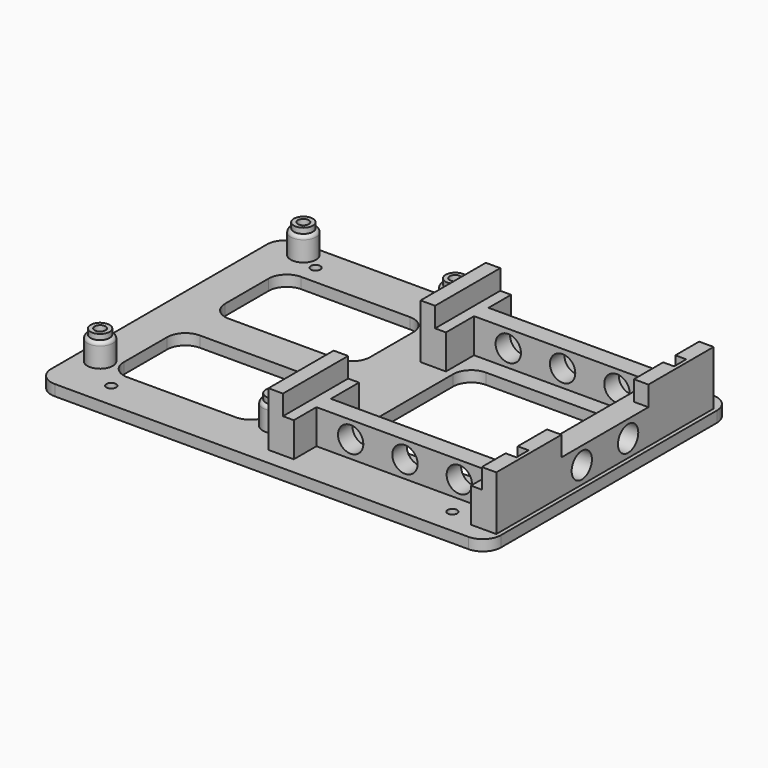
from build123d import *

# Parameters (mm, degrees)
F0_R      = 1.325
F1_DEPTH  = 3
F2_R      = 2.625
F2_R_2    = 1.5
F3_DEPTH  = 8
F4_R      = 3.5
F5_DEPTH  = 6.5
F7_DEPTH  = 7.5
F8_W      = 4
F8_H      = 75
F9_DEPTH  = 10
F10_W     = 4
F10_H     = 75
F11_DEPTH = 10
F13_DEPTH = 10
F14_W     = 30
F14_H     = 17.5
F15_DEPTH = 64.001
F16_W     = 4
F16_H     = 2.5
F17_DEPTH = 79.751
F20_DEPTH = 3.001
F18_W     = 48.9
F18_H     = 5
F21_DEPTH = 7.5
F23_DEPTH = 3.001
F24_W     = 4
F24_H     = 2.5
F25_DEPTH = 79.751
F26_DEPTH = 9.501
F27_W     = 7
F27_H     = 30
F28_DEPTH = 7.5
F30_DEPTH = 2
F31_R     = 3.5
F32_DEPTH = 71.951
F33_R     = 3.5
F34_DEPTH = 123.101


# Not quite as in the source:
# - a fillet or chamfer that OpenCascade refuses, or shapes differently, is made with other operations: its cross-section is extruded or revolved along the edge and cut away or added


with BuildPart() as f1:
    # F0 (on Top) → F1 (new body)
    with BuildSketch(Plane.XY):
        with BuildLine():
            Line((57.1, 42.25), (0, 42.25))
            Line((0, 42.25), (-57.1, 42.25))
            ThreePointArc((-57.1, 42.25), (-60.6355339059, 40.7855339059), (-62.1, 37.25))
            Line((-62.1, 37.25), (-62.1, 0))
            Line((-62.1, 0), (-62.1, -37.25))
            ThreePointArc((-62.1, -37.25), (-60.6355339059, -40.7855339059), (-57.1, -42.25))
            Line((-57.1, -42.25), (0, -42.25))
            Line((0, -42.25), (57.1, -42.25))
            ThreePointArc((57.1, -42.25), (60.6355339059, -40.7855339059), (62.1, -37.25))
            Line((62.1, -37.25), (62.1, 0))
            Line((62.1, 0), (62.1, 37.25))
            ThreePointArc((62.1, 37.25), (60.6355339059, 40.7855339059), (57.1, 42.25))
        make_face()
        with Locations((-47.1, -35.25)):
            Circle(F0_R, mode=Mode.SUBTRACT)
        with Locations((47.1, -35.25)):
            Circle(F0_R, mode=Mode.SUBTRACT)
        with Locations((-47.1, 35.25)):
            Circle(F0_R, mode=Mode.SUBTRACT)
        with Locations((47.1, 35.25)):
            Circle(F0_R, mode=Mode.SUBTRACT)
    extrude(amount=F1_DEPTH)

    # F2 (on face) → F3 (join)
    with BuildSketch(Plane.XY.offset(3)):
        with Locations((-56.1, -27.85)):
            Circle(F2_R)
        with Locations((-56.1, -27.85)):
            Circle(F2_R_2, mode=Mode.SUBTRACT)
        with Locations((-7.71, -27.85)):
            Circle(F2_R)
        with Locations((-7.71, -27.85)):
            Circle(F2_R_2, mode=Mode.SUBTRACT)
        with Locations((-52.86, 38.25)):
            Circle(F2_R)
        with Locations((-52.86, 38.25)):
            Circle(F2_R_2, mode=Mode.SUBTRACT)
        with Locations((-10.95, 38.25)):
            Circle(F2_R)
        with Locations((-10.95, 38.25)):
            Circle(F2_R_2, mode=Mode.SUBTRACT)
    extrude(amount=F3_DEPTH)

    # F4 (on face) → F5 (join)
    with BuildSketch(Plane.XY.offset(3)):
        with Locations((-10.95, 38.25)):
            Circle(F4_R)
        with Locations((-7.71, -27.85)):
            Circle(F4_R)
        with Locations((-56.1, -27.85)):
            Circle(F4_R)
        with Locations((-52.86, 38.25)):
            Circle(F4_R)
    extrude(amount=F5_DEPTH)

    # F6 (on face) → F7 (join)
    with BuildSketch(Plane.XY.offset(3)):
        Polygon((5.1, 37.5), (2.1, 37.5), (-1.9, 37.5), (-1.9, -37.5), (2.1, -37.5), (5.1, -37.5), align=None)
        Polygon((61, 37.5), (57, 37.5), (54, 37.5), (54, -37.5), (57, -37.5), (61, -37.5), align=None)
    extrude(amount=F7_DEPTH)

    # F8 (on face) → F9 (join)
    with BuildSketch(Plane.XY.offset(10.5)):
        with Locations((0.1, 0)):
            Rectangle(F8_W, F8_H)
    extrude(amount=F9_DEPTH)

    # F10 (on face) → F11 (join)
    with BuildSketch(Plane.XY.offset(10.5)):
        with Locations((59, 0)):
            Rectangle(F10_W, F10_H)
    extrude(amount=F11_DEPTH)

    # F12 (on face) → F13 (cut)
    with BuildSketch(Plane.XY.offset(20.5)):
        Polygon((60, -25.1), (57, -25.1), (57, -29.3), (60, -29.3), (60, -27.2), align=None)
        Polygon((60, 27.2), (60, 29.3), (57, 29.3), (57, 25.1), (60, 25.1), align=None)
    extrude(amount=-F13_DEPTH, mode=Mode.SUBTRACT)

    # F14 (on face) → F15 (cut, through all)
    with BuildSketch(Plane(origin=(-1.9, 0, 0), x_dir=(0, -1, 0), z_dir=(-1, 0, 0))):
        with Locations((0, 11.75)):
            Rectangle(F14_W, F14_H)
    extrude(amount=-F15_DEPTH, mode=Mode.SUBTRACT)

    # F16 (on face) → F17 (cut, through all)
    with BuildSketch(Plane.XZ.offset(37.5)):
        with Locations((0.1, 19.25)):
            Rectangle(F16_W, F16_H)
    extrude(amount=-F17_DEPTH, mode=Mode.SUBTRACT)

    # F19 (on face) → F20 (cut, through all)
    with BuildSketch(Plane.XY.offset(3)):
        with BuildLine():
            Line((47.1, 20), (12.1, 20))
            ThreePointArc((12.1, 20), (8.5644660941, 18.5355339059), (7.1, 15))
            Line((7.1, 15), (7.1, -15))
            ThreePointArc((7.1, -15), (8.5644660941, -18.5355339059), (12.1, -20))
            Line((12.1, -20), (47.1, -20))
            ThreePointArc((47.1, -20), (50.6355339059, -18.5355339059), (52.1, -15))
            Line((52.1, -15), (52.1, 15))
            ThreePointArc((52.1, 15), (50.6355339059, 18.5355339059), (47.1, 20))
        make_face()
    extrude(amount=-F20_DEPTH, mode=Mode.SUBTRACT)

    # F18 (on face) → F21 (join)
    with BuildSketch(Plane.XY.offset(3)):
        with Locations((29.55, -27.2)):
            Rectangle(F18_W, F18_H)
        with Locations((29.55, 27.2)):
            Rectangle(F18_W, F18_H)
    extrude(amount=F21_DEPTH)

    # F22 (on face) → F23 (cut, through all)
    with BuildSketch(Plane.XY.offset(3)):
        with BuildLine():
            Line((-16.85, 30), (-46.85, 30))
            ThreePointArc((-46.85, 30), (-50.3855339059, 28.5355339059), (-51.85, 25))
            Line((-51.85, 25), (-51.85, 10))
            ThreePointArc((-51.85, 10), (-50.3855339059, 6.4644660941), (-46.85, 5))
            Line((-46.85, 5), (-16.85, 5))
            ThreePointArc((-16.85, 5), (-13.3144660941, 6.4644660941), (-11.85, 10))
            Line((-11.85, 10), (-11.85, 25))
            ThreePointArc((-11.85, 25), (-13.3144660941, 28.5355339059), (-16.85, 30))
        make_face()
        with BuildLine():
            Line((-46.85, -30), (-16.85, -30))
            ThreePointArc((-16.85, -30), (-13.3144660941, -28.5355339059), (-11.85, -25))
            Line((-11.85, -25), (-11.85, -10))
            ThreePointArc((-11.85, -10), (-13.3144660941, -6.4644660941), (-16.85, -5))
            Line((-16.85, -5), (-46.85, -5))
            ThreePointArc((-46.85, -5), (-50.3855339059, -6.4644660941), (-51.85, -10))
            Line((-51.85, -10), (-51.85, -25))
            ThreePointArc((-51.85, -25), (-50.3855339059, -28.5355339059), (-46.85, -30))
        make_face()
    extrude(amount=-F23_DEPTH, mode=Mode.SUBTRACT)

    # F24 (on face) → F25 (cut, through all)
    with BuildSketch(Plane.XZ.offset(37.5)):
        with Locations((59, 19.25)):
            Rectangle(F24_W, F24_H)
    extrude(amount=-F25_DEPTH, mode=Mode.SUBTRACT)

    # F26 (cut, through all): faces of the model
    f26_faces = [f1.faces().sort_by_distance(p)[0] for p in [
        (-52.86, 38.25, 9.5),
        (-10.95, 38.25, 9.5),
        (-7.71, -27.85, 9.5),
        (-56.1, -27.85, 9.5),
    ]]
    extrude(f26_faces, amount=-F26_DEPTH, mode=Mode.SUBTRACT)

    # F27 (on face) → F28 (join)
    with BuildSketch(Plane.XY.offset(3)):
        with Locations((57.5, 0)):
            Rectangle(F27_W, F27_H)
    extrude(amount=F28_DEPTH)

    # F29: fillet of radius 1 on 4 edges, made by hand

    # F29_s1 → F29_t2 (revolve, cut)
    with BuildSketch(Plane.XZ.offset(-38.25)):
        with BuildLine():
            ThreePointArc((-49.36, 8.5078432584), (-49.61, 9.1692810861), (-50.235, 9.5))
            Line((-50.235, 9.5), (-49.36, 9.5))
            Line((-49.36, 9.5), (-49.36, 8.5078432584))
        make_face()
    revolve(axis=Axis((-52.86, 38.25, 9.5), (0, 0, 1)), mode=Mode.SUBTRACT)

    # F29_s3 → F29_t4 (revolve, cut)
    with BuildSketch(Plane.XZ.offset(-38.25)):
        with BuildLine():
            ThreePointArc((-7.45, 8.5078432584), (-7.7, 9.1692810861), (-8.325, 9.5))
            Line((-8.325, 9.5), (-7.45, 9.5))
            Line((-7.45, 9.5), (-7.45, 8.5078432584))
        make_face()
    revolve(axis=Axis((-10.95, 38.25, 9.5), (0, 0, 1)), mode=Mode.SUBTRACT)

    # F29_s5 → F29_t6 (revolve, cut)
    with BuildSketch(Plane.XZ.offset(27.85)):
        with BuildLine():
            ThreePointArc((-4.21, 8.5078432584), (-4.46, 9.1692810861), (-5.085, 9.5))
            Line((-5.085, 9.5), (-4.21, 9.5))
            Line((-4.21, 9.5), (-4.21, 8.5078432584))
        make_face()
    revolve(axis=Axis((-7.71, -27.85, 9.5), (0, 0, 1)), mode=Mode.SUBTRACT)

    # F29_s7 → F29_t8 (revolve, cut)
    with BuildSketch(Plane.XZ.offset(27.85)):
        with BuildLine():
            ThreePointArc((-52.6, 8.5078432584), (-52.85, 9.1692810861), (-53.475, 9.5))
            Line((-53.475, 9.5), (-52.6, 9.5))
            Line((-52.6, 9.5), (-52.6, 8.5078432584))
        make_face()
    revolve(axis=Axis((-56.1, -27.85, 9.5), (0, 0, 1)), mode=Mode.SUBTRACT)

    # F30 (add): a face of the model
    f30_faces = [f1.faces().sort_by_distance(p)[0] for p in [
        (3.6, -36.5463643253, 10.5),
    ]]
    extrude(f30_faces, amount=F30_DEPTH)

    # F31 (on face) → F32 (cut, through all)
    with BuildSketch(Plane.XZ.offset(29.7)):
        with Locations((29.55, 7.75)):
            Circle(F31_R)
        with Locations((14.55, 7.75)):
            Circle(F31_R)
        with Locations((44.55, 7.75)):
            Circle(F31_R)
    extrude(amount=-F32_DEPTH, mode=Mode.SUBTRACT)

    # F33 (on face) → F34 (cut, through all)
    with BuildSketch(Plane.YZ.offset(61)):
        with Locations((-8, 7.75)):
            Circle(F33_R)
        with Locations((8, 7.75)):
            Circle(F33_R)
    extrude(amount=-F34_DEPTH, mode=Mode.SUBTRACT)


solid = f1.part
